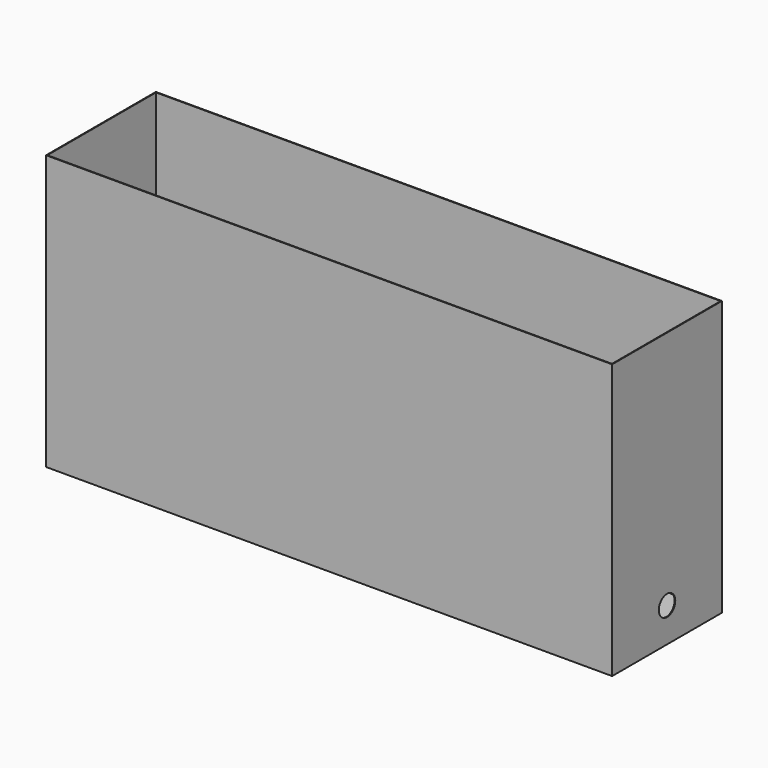
from build123d import *

# Parameters (mm, degrees)
F0_W     = 825
F0_H     = 200
F1_DEPTH = 400
F2_T     = -1
F5_D     = 40
F7_D     = 30


# Not quite as in the source:
# - the program builds the solid bodies; features that only make, move or delete a surface that nothing else refers to are left out


with BuildPart() as f1:
    # F0 (on Top) → F1 (new body)
    with BuildSketch(Plane.XY):
        Rectangle(F0_W, F0_H)
    extrude(amount=F1_DEPTH)

    # F2
    f2_openings = [f1.faces().sort_by_distance(p)[0] for p in [
        (0, 0, 400),
    ]]
    offset(amount=F2_T, openings=f2_openings)

    # F5 (through all)
    with Locations(Plane.XY.offset(1)):
        with Locations((389.5, 77), (389.5, -77), (-389.5, 77), (-389.5, -77)):
            Hole(F5_D / 2)

    # F7 (through all)
    with Locations(Plane(origin=(-412.5, 0, 0), x_dir=(0, -1, 0), z_dir=(-1, 0, 0))):
        with Locations((0, 50)):
            Hole(F7_D / 2)


solid = f1.part
